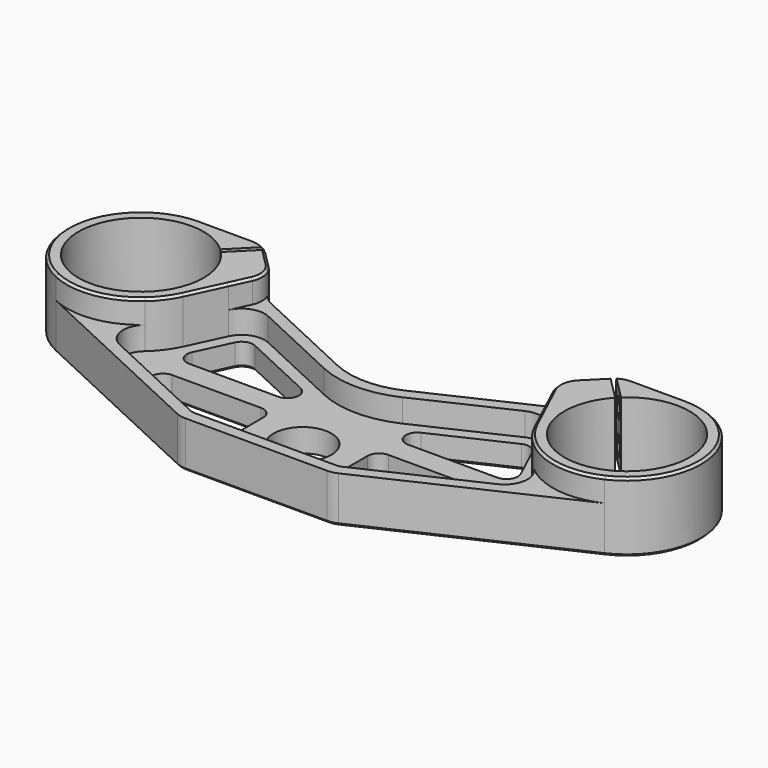
from build123d import *

# Parameters (mm, degrees)
F1_DEPTH = 30
F0_R     = 12.5
F2_DEPTH = 10
F3_DEPTH = 20
F4_SIZE  = 1
F6_START = 6
F5_R     = 6.75
F5_R_2   = 4.2
F5_R_3   = 7.125
F6_DEPTH = 16
F7_DEPTH = 25
F8_D     = 6.8
F8_DEPTH = 15.75
F8_TIP   = 2.0429261047


with BuildPart() as f1:
    # F0 (on Top) → F1 (new body)
    with BuildSketch(Plane.XY):
        with BuildLine():
            ThreePointArc((66.9448760651, 65.3418456847), (65.9895686562, 64.2354489297), (65.2057628955, 63.0016034958))
            ThreePointArc((65.2057628955, 63.0016034958), (64.0199274379, 58.5530106666), (64.9528660066, 54.0445952555))
            Line((64.9528660066, 54.0445952555), (68.7471940628, 45.9076324802))
            Line((68.7471940628, 45.9076324802), (75.9528354255, 30.4550847112))
            ThreePointArc((75.9528354255, 30.4550847112), (79.3903671328, 24.7295769531), (83.9397925791, 19.8407333847))
            ThreePointArc((83.9397925791, 19.8407333847), (100.5175017487, 12.2650081231), (118.5449152888, 14.9528354255))
            ThreePointArc((118.5449152888, 14.9528354255), (136.2902870282, 50.9368896267), (105, 76.05))
            Line((105, 76.05), (81.7951660041, 76.05))
            ThreePointArc((81.7951660041, 76.05), (78.8269511444, 75.599329848), (76.126273453, 74.2879401093))
            Line((76.126273453, 74.2879401093), (86.5929431845, 63.8212703778))
            ThreePointArc((86.5929431845, 63.8212703778), (124.1272384311, 24.8727615689), (85.1787296222, 62.4070568155))
            Line((85.1787296222, 62.4070568155), (74.594408409, 72.9913780286))
            Line((74.594408409, 72.9913780286), (66.9448760651, 65.3418456847))
        make_face()
    extrude(amount=F1_DEPTH)



with BuildPart() as f1b:
    # F0 (on Top) → F1, piece 2 (new body)
    with BuildSketch(Plane.XY):
        with BuildLine():
            ThreePointArc((-85.1787296222, 62.4070568155), (-124.1272384311, 24.8727615689), (-86.5929431845, 63.8212703778))
            Line((-86.5929431845, 63.8212703778), (-76.126273453, 74.2879401093))
            ThreePointArc((-76.126273453, 74.2879401093), (-78.8269511444, 75.599329848), (-81.7951660041, 76.05))
            Line((-81.7951660041, 76.05), (-105, 76.05))
            ThreePointArc((-105, 76.05), (-136.2902869122, 50.9368901498), (-118.54491626, 14.9528358783))
            ThreePointArc((-118.54491626, 14.9528358783), (-100.5175022793, 12.2650080482), (-83.9397925791, 19.8407333847))
            ThreePointArc((-83.9397925791, 19.8407333847), (-79.3903671328, 24.7295769531), (-75.9528354255, 30.4550847112))
            Line((-75.9528354255, 30.4550847112), (-68.7471940628, 45.9076324802))
            Line((-68.7471940628, 45.9076324802), (-64.9528660066, 54.0445952555))
            ThreePointArc((-64.9528660066, 54.0445952555), (-64.0199274379, 58.5530106666), (-65.2057628955, 63.0016034958))
            ThreePointArc((-65.2057628955, 63.0016034958), (-65.9895686562, 64.2354489297), (-66.9448760651, 65.3418456847))
            Line((-66.9448760651, 65.3418456847), (-74.594408409, 72.9913780286))
            Line((-74.594408409, 72.9913780286), (-85.1787296222, 62.4070568155))
        make_face()
    extrude(amount=F1_DEPTH)


with BuildPart() as f1_1:
    add(f1.part)

    add(f1b.part)  # F2 merges F1b
    # F0 (on Top) → F2 (join)
    with BuildSketch(Plane.XY):
        with BuildLine():
            ThreePointArc((-75.9528354255, 30.4550847112), (-79.3903671328, 24.7295769531), (-83.9397925791, 19.8407333847))
            ThreePointArc((-83.9397925791, 19.8407333847), (-87.2704585561, 10.9041452828), (-81.5949276393, 3.2396628106))
            Line((-81.5949276393, 3.2396628106), (-32.7619279072, -19.5315389352))
            ThreePointArc((-32.7619279072, -19.5315389352), (-31.7310346681, -19.8814800356), (-30.6488365984, -20))
            Line((-30.6488365984, -20), (30.6488365984, -20))
            ThreePointArc((30.6488365984, -20), (31.7310346681, -19.8814800356), (32.7619279072, -19.5315389352))
            Line((32.7619279072, -19.5315389352), (81.5949276393, 3.2396628106))
            ThreePointArc((81.5949276393, 3.2396628106), (87.2704585561, 10.9041452828), (83.9397925791, 19.8407333847))
            ThreePointArc((83.9397925791, 19.8407333847), (79.3903671328, 24.7295769531), (75.9528354255, 30.4550847112))
            Line((75.9528354255, 30.4550847112), (68.7471940628, 45.9076324802))
            ThreePointArc((68.7471940628, 45.9076324802), (63.1043176257, 51.0783760706), (55.457933575, 50.7445277331))
            Line((55.457933575, 50.7445277331), (16.9047304696, 32.7668738787))
            ThreePointArc((16.9047304696, 32.7668738787), (0, 29.0191853602), (-16.9047304696, 32.7668738787))
            Line((-16.9047304696, 32.7668738787), (-55.457933575, 50.7445277331))
            ThreePointArc((-55.457933575, 50.7445277331), (-63.1043176257, 51.0783760706), (-68.7471940628, 45.9076324802))
            Line((-68.7471940628, 45.9076324802), (-75.9528354255, 30.4550847112))
        make_face()
        with BuildLine():
            Line((-29.6130913087, -15.4829759605), (-68.0028468966, 2.4184610648))
            ThreePointArc((-68.0028468966, 2.4184610648), (-70.7712356235, 8.0321980697), (-65.8897555879, 11.95))
            Line((-65.8897555879, 11.95), (-27.5, 11.95))
            ThreePointArc((-27.5, 11.95), (-23.9644660941, 10.4855339059), (-22.5, 6.95))
            Line((-22.5, 6.95), (-22.5, -10.9514370253))
            ThreePointArc((-22.5, -10.9514370253), (-24.8135019583, -15.1683942544), (-29.6130913087, -15.4829759605))
        make_face(mode=Mode.SUBTRACT)
        Circle(F0_R, mode=Mode.SUBTRACT)
        with BuildLine():
            ThreePointArc((65.8897555879, 11.95), (70.7712356235, 8.0321980697), (68.0028468966, 2.4184610648))
            Line((68.0028468966, 2.4184610648), (29.6130913087, -15.4829759605))
            ThreePointArc((29.6130913087, -15.4829759605), (24.8135019583, -15.1683942544), (22.5, -10.9514370253))
            Line((22.5, -10.9514370253), (22.5, 6.95))
            ThreePointArc((22.5, 6.95), (23.9644660941, 10.4855339059), (27.5, 11.95))
            Line((27.5, 11.95), (65.8897555879, 11.95))
        make_face(mode=Mode.SUBTRACT)
        with BuildLine():
            Line((-28.0924200126, 21.95), (-66.5535040792, 21.95))
            ThreePointArc((-66.5535040792, 21.95), (-70.7704613082, 24.2635019583), (-71.0850430144, 29.0630913087))
            Line((-71.0850430144, 29.0630913087), (-64.2156551276, 43.7945411715))
            ThreePointArc((-64.2156551276, 43.7945411715), (-61.3942169091, 46.3799129667), (-57.5710248837, 46.212988798))
            Line((-57.5710248837, 46.212988798), (-25.9793287039, 31.4815389352))
            ThreePointArc((-25.9793287039, 31.4815389352), (-23.210939977, 25.8678019303), (-28.0924200126, 21.95))
        make_face(mode=Mode.SUBTRACT)
        with BuildLine():
            Line((25.9793287039, 31.4815389352), (57.5710248837, 46.212988798))
            ThreePointArc((57.5710248837, 46.212988798), (61.3942169091, 46.3799129667), (64.2156551276, 43.7945411715))
            Line((64.2156551276, 43.7945411715), (71.0850430144, 29.0630913087))
            ThreePointArc((71.0850430144, 29.0630913087), (70.7704613082, 24.2635019583), (66.5535040792, 21.95))
            Line((66.5535040792, 21.95), (28.0924200126, 21.95))
            ThreePointArc((28.0924200126, 21.95), (23.210939977, 25.8678019303), (25.9793287039, 31.4815389352))
        make_face(mode=Mode.SUBTRACT)
    extrude(amount=F2_DEPTH)

    # F0 (on Top) → F3 (join)
    with BuildSketch(Plane.XY):
        with BuildLine():
            ThreePointArc((-60.6217645315, 58.6693512484), (-63.2642642007, 60.4646093875), (-65.2057628955, 63.0016034958))
            ThreePointArc((-65.2057628955, 63.0016034958), (-64.0199274379, 58.5530106666), (-64.9528660066, 54.0445952555))
            Line((-64.9528660066, 54.0445952555), (-68.7471940628, 45.9076324802))
            ThreePointArc((-68.7471940628, 45.9076324802), (-63.1043176257, 51.0783760706), (-55.457933575, 50.7445277331))
            Line((-55.457933575, 50.7445277331), (-16.9047304696, 32.7668738787))
            ThreePointArc((-16.9047304696, 32.7668738787), (0, 29.0191853602), (16.9047304696, 32.7668738787))
            Line((16.9047304696, 32.7668738787), (55.457933575, 50.7445277331))
            ThreePointArc((55.457933575, 50.7445277331), (63.1043176257, 51.0783760706), (68.7471940628, 45.9076324802))
            Line((68.7471940628, 45.9076324802), (64.9528660066, 54.0445952555))
            ThreePointArc((64.9528660066, 54.0445952555), (64.0199274379, 58.5530106666), (65.2057628955, 63.0016034958))
            ThreePointArc((65.2057628955, 63.0016034958), (63.2642642007, 60.4646093875), (60.6217645315, 58.6693512484))
            Line((60.6217645315, 58.6693512484), (14.7916391609, 37.2984128139))
            ThreePointArc((14.7916391609, 37.2984128139), (0, 34.0191853602), (-14.7916391609, 37.2984128139))
            Line((-14.7916391609, 37.2984128139), (-60.6217645315, 58.6693512484))
        make_face()
        with BuildLine():
            ThreePointArc((-83.9397925791, 19.8407333847), (-100.5175022793, 12.2650080482), (-118.54491626, 14.9528358783))
            Line((-118.54491626, 14.9528358783), (-34.8750192159, -24.0630778704))
            ThreePointArc((-34.8750192159, -24.0630778704), (-32.8132327378, -24.7629600712), (-30.6488365984, -25))
            Line((-30.6488365984, -25), (30.6488365984, -25))
            ThreePointArc((30.6488365984, -25), (32.8132327378, -24.7629600712), (34.8750192159, -24.0630778704))
            Line((34.8750192159, -24.0630778704), (118.5449152888, 14.9528354255))
            ThreePointArc((118.5449152888, 14.9528354255), (100.5175017487, 12.2650081231), (83.9397925791, 19.8407333847))
            ThreePointArc((83.9397925791, 19.8407333847), (87.2704585561, 10.9041452828), (81.5949276393, 3.2396628106))
            Line((81.5949276393, 3.2396628106), (32.7619279072, -19.5315389352))
            ThreePointArc((32.7619279072, -19.5315389352), (31.7310346681, -19.8814800356), (30.6488365984, -20))
            Line((30.6488365984, -20), (-30.6488365984, -20))
            ThreePointArc((-30.6488365984, -20), (-31.7310346681, -19.8814800356), (-32.7619279072, -19.5315389352))
            Line((-32.7619279072, -19.5315389352), (-81.5949276393, 3.2396628106))
            ThreePointArc((-81.5949276393, 3.2396628106), (-87.2704585561, 10.9041452828), (-83.9397925791, 19.8407333847))
        make_face()
    extrude(amount=F3_DEPTH)

    # F4
    f4_edges = [f1_1.edges().sort_by_distance(p)[0] for p in [
        (-76.709968, -4.555121, 0),
        (-136.290287, 50.93689, 0),
        (-37.706702, 47.983882, 0),
        (48.807969, -6.532257, 0),
        (47.322962, 21.95, 0),
        (-41.775177, 38.847264, 0),
        (-46.694878, 11.95, 0),
        (132.030696, 26.779548, 30),
        (-70.769642, 69.166612, 0),
        (-93.397583, 76.05, 30),
        (-70.452851, 42.24984, 30),
        (-65.989569, 64.235449, 0),
        (-64.167866, 60.00726, 30),
        (-70.769642, 69.166612, 30),
        (-78.826951, 75.59933, 30),
        (-135.012556, 32.755045, 30),
        (-79.390367, 24.729577, 30),
        (0, 34.019185, 0),
        (-63.264264, 60.464609, 0),
        (70.452851, 42.24984, 30),
        (65.989569, 64.235449, 0),
        (64.167866, 60.00726, 30),
        (63.264264, 60.464609, 0),
        (37.706702, 47.983882, 0),
        (-78.826951, 75.59933, 0),
        (-93.397583, 76.05, 0),
        (-32.813233, -24.76296, 0),
        (0, -25, 0),
        (32.813233, -24.76296, 0),
        (76.709967, -4.555121, 0),
        (136.290287, 50.93689, 0),
        (93.397583, 76.05, 0),
        (78.826951, 75.59933, 0),
        (70.769642, 69.166612, 0),
        (-23.21094, 25.867802, 0),
        (-47.322962, 21.95, 0),
        (-70.770461, 24.263502, 0),
        (-67.650349, 36.428816, 0),
        (-61.394217, 46.379913, 0),
        (23.21094, 25.867802, 0),
        (41.775177, 38.847264, 0),
        (61.394217, 46.379913, 0),
        (67.650349, 36.428816, 0),
        (70.770461, 24.263502, 0),
        (-48.807969, -6.532257, 0),
        (-70.771236, 8.032198, 0),
        (-23.964466, 10.485534, 0),
        (-22.5, -2.000719, 0),
        (-24.813502, -15.168394, 0),
        (70.771236, 8.032198, 0),
        (24.813502, -15.168394, 0),
        (22.5, -2.000719, 0),
        (23.964466, 10.485534, 0),
        (46.694878, 11.95, 0),
        (93.397583, 76.05, 30),
        (78.826951, 75.59933, 30),
        (70.769642, 69.166612, 30),
    ]]
    chamfer(f4_edges, length=F4_SIZE)

    # F5 (on face) → F6 (cut)
    with BuildSketch(Plane(origin=(73.7928932188, 73.7928932188, 0), x_dir=(-0.7071067812, 0.7071067812, 0), z_dir=(0.7071067812, 0.7071067812, 0)).offset(F6_START)):
        with Locations((-8.6177589565, 7.75)):
            Circle(F5_R)
        with Locations((-8.6177589565, 7.75)):
            Circle(F5_R_2, mode=Mode.SUBTRACT)
        with Locations((-8.6177589565, 22.25)):
            Circle(F5_R_3)
        with Locations((-8.6177589565, 22.25)):
            Circle(F5_R_2, mode=Mode.SUBTRACT)
        with Locations((-8.6177589565, 22.25)):
            Circle(F5_R_2)
        with Locations((-8.6177589565, 7.75)):
            Circle(F5_R_2)
    extrude(amount=F6_DEPTH, mode=Mode.SUBTRACT)

    # F5 (on face) → F7 (cut)
    with BuildSketch(Plane(origin=(73.7928932188, 73.7928932188, 0), x_dir=(-0.7071067812, 0.7071067812, 0), z_dir=(0.7071067812, 0.7071067812, 0))):
        with Locations((-8.6177589565, 7.75)):
            Circle(F5_R_2)
        with Locations((-8.6177589565, 22.25)):
            Circle(F5_R_2)
    extrude(amount=F7_DEPTH, mode=Mode.SUBTRACT)

    # F8
    with Locations(Plane(origin=(73.7928932188, 73.7928932188, 0), x_dir=(-0.7071067812, 0.7071067812, 0), z_dir=(0.7071067812, 0.7071067812, 0))):
        with Locations((-8.6177589565, 7.75), (-8.6177589565, 22.25)):
            Hole(F8_D / 2, depth=F8_DEPTH)
            with Locations((0, 0, -(F8_DEPTH + F8_TIP / 2))):  # 118° drill point
                Cone(0, F8_D / 2, F8_TIP, mode=Mode.SUBTRACT)


solid = f1_1.part
